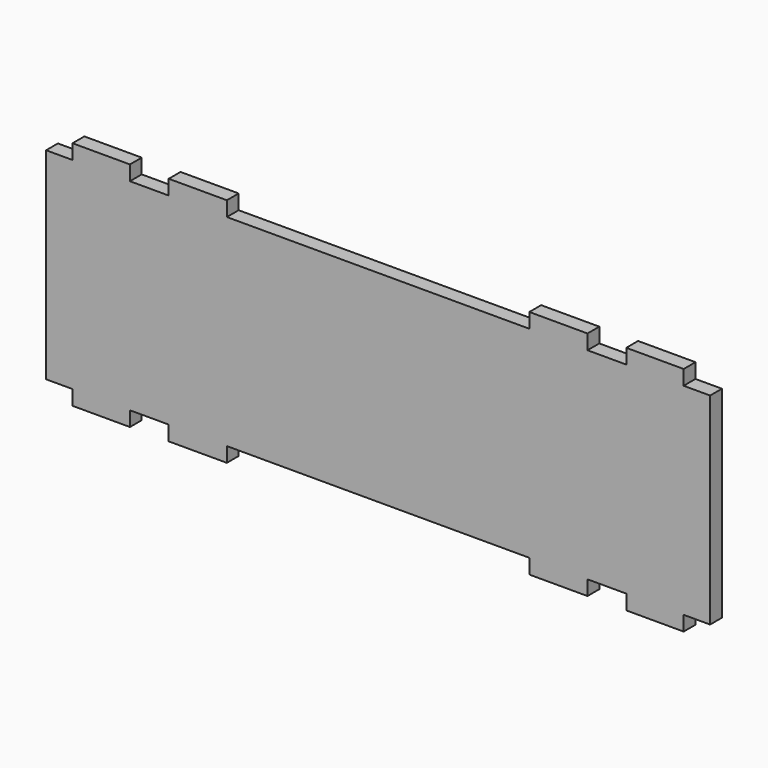
from build123d import *

# Parameters (mm, degrees)
F0_W     = 14.8
F0_H     = 3.81
F0_W_2   = 15
F1_DEPTH = 3.81


# Not quite as in the source:
# - a feature names something its author has since deleted; it is built from what else it names


with BuildPart() as f1:
    # F0 (on Front) → F1 (new body)
    with BuildSketch(Plane.XZ):
        Polygon((85.62, 0), (85.62, 26), (78.8, 26), (64, 26), (54, 26), (39, 26), (0, 26), (0, 0), align=None)
        Polygon((-85.62, 0), (0, 0), (0, 26), (-39, 26), (-54, 26), (-64, 26), (-78.8, 26), (-85.62, 26), align=None)
        Polygon((0, -26), (0, 0), (-85.62, 0), (-85.62, -26), (-78.8, -26), (-64, -26), (-54, -26), (-39, -26), align=None)
        Polygon((85.62, -26), (85.62, 0), (0, 0), (0, -26), (39, -26), (54, -26), (64, -26), (78.8, -26), align=None)
        with Locations((71.4, 27.905)):
            Rectangle(F0_W, F0_H)
        with Locations((-71.4, -27.905)):
            Rectangle(F0_W, F0_H)
        with Locations((-71.4, 27.905)):
            Rectangle(F0_W, F0_H)
        with Locations((71.4, -27.905)):
            Rectangle(F0_W, F0_H)
        with Locations((-46.5, 27.905)):
            Rectangle(F0_W_2, F0_H)
        with Locations((-46.5, -27.905)):
            Rectangle(F0_W_2, F0_H)
        with Locations((46.5, -27.905)):
            Rectangle(F0_W_2, F0_H)
        with Locations((46.5, 27.905)):
            Rectangle(F0_W_2, F0_H)
    extrude(amount=F1_DEPTH)


solid = f1.part
